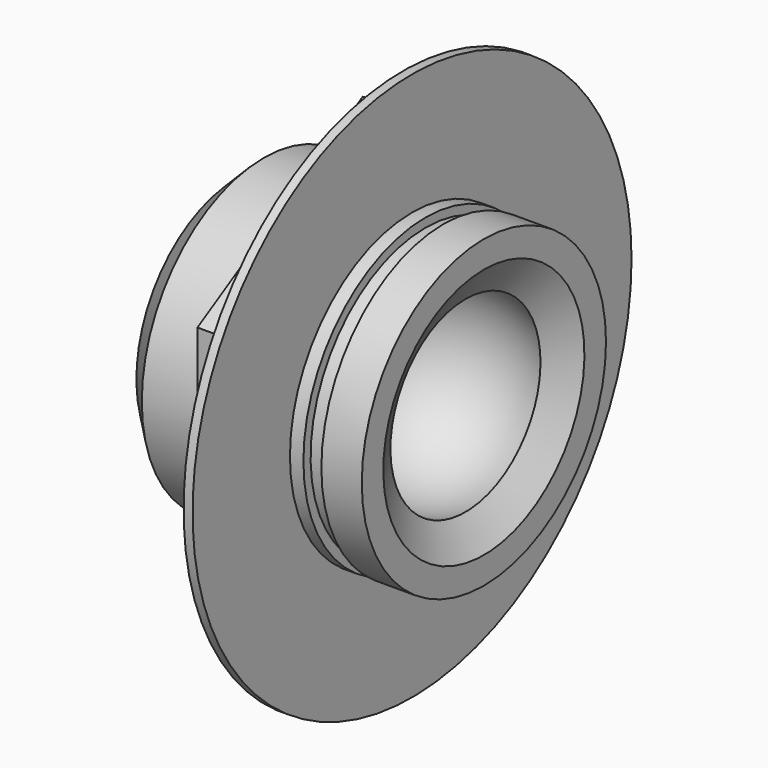
from build123d import *

# Parameters (mm, degrees)
F3_DEPTH = 25
F4_SIZE  = 3
F5_R     = 30.5581123827
F5_R_2   = 17
F6_DEPTH = 1


with BuildPart() as f1:
    # F0 (on Front) → F1 (revolve)
    with BuildSketch(Plane.XZ):
        with BuildLine():
            Line((0, 17), (0, 0))
            Line((0, 0), (11, 0))
            ThreePointArc((11, 0), (15.5551164444, 8.914228848), (25.4479047191, 10.4456667115))
            Line((25.4479047191, 10.4456667115), (27.5, 14))
            Line((27.5, 14), (27.5, 17))
            Line((27.5, 17), (23, 17))
            Line((23, 17), (23, 16))
            Line((23, 16), (21, 16))
            Line((21, 16), (21, 17))
            Line((21, 17), (18.5, 17))
            Line((18.5, 17), (18.5, 40))
            Line((18.5, 40), (14, 40))
            Line((14, 40), (14, 17))
            Line((14, 17), (0, 17))
        make_face()
    revolve(axis=Axis((11, 0, 0), (1, 0, 0)))

    # F2 (on face) → F3 (cut)
    with BuildSketch(Plane(origin=(14, 0, 0), x_dir=(0, -1, 0), z_dir=(-1, 0, 0))):
        with BuildLine():
            ThreePointArc((16.8416654415, -36.281652459), (20, -34.6410161514), (23, -32.7261363439))
            Line((23, -32.7261363439), (23, -13.2790561914))
            Line((23, -13.2790561914), (0, -26.5581123827))
            Line((0, -26.5581123827), (16.8416654415, -36.281652459))
        make_face()
        with BuildLine():
            Line((23, -13.2790561914), (23, -32.7261363439))
            ThreePointArc((23, -32.7261363439), (34.6410161514, -20), (39.8416654415, -3.5555161151))
            Line((39.8416654415, -3.5555161151), (23, -13.2790561914))
        make_face()
        with BuildLine():
            Line((23, 13.2790561914), (23, -13.2790561914))
            Line((23, -13.2790561914), (39.8416654415, -3.5555161151))
            ThreePointArc((39.8416654415, -3.5555161151), (39.9603967552, -1.7795199266), (40, 0))
            ThreePointArc((40, 0), (39.9603967552, 1.7795199266), (39.8416654415, 3.5555161151))
            Line((39.8416654415, 3.5555161151), (23, 13.2790561914))
        make_face()
        with BuildLine():
            Line((23, 32.7261363439), (23, 13.2790561914))
            Line((23, 13.2790561914), (39.8416654415, 3.5555161151))
            ThreePointArc((39.8416654415, 3.5555161151), (34.6410161514, 20), (23, 32.7261363439))
        make_face()
        with BuildLine():
            Line((0, 26.5581123827), (23, 13.2790561914))
            Line((23, 13.2790561914), (23, 32.7261363439))
            ThreePointArc((23, 32.7261363439), (20, 34.6410161514), (16.8416654415, 36.281652459))
            Line((16.8416654415, 36.281652459), (0, 26.5581123827))
        make_face()
        with BuildLine():
            Line((-16.8416654415, 36.281652459), (0, 26.5581123827))
            Line((0, 26.5581123827), (16.8416654415, 36.281652459))
            ThreePointArc((16.8416654415, 36.281652459), (0, 40), (-16.8416654415, 36.281652459))
        make_face()
        with BuildLine():
            Line((-23, 13.2790561914), (0, 26.5581123827))
            Line((0, 26.5581123827), (-16.8416654415, 36.281652459))
            ThreePointArc((-16.8416654415, 36.281652459), (-20, 34.6410161514), (-23, 32.7261363439))
            Line((-23, 32.7261363439), (-23, 13.2790561914))
        make_face()
        with BuildLine():
            Line((-39.8416654415, -3.5555161151), (-23, -13.2790561914))
            Line((-23, -13.2790561914), (-23, 13.2790561914))
            Line((-23, 13.2790561914), (-39.8416654415, 3.5555161151))
            ThreePointArc((-39.8416654415, 3.5555161151), (-40, 0), (-39.8416654415, -3.5555161151))
        make_face()
        with BuildLine():
            Line((-23, -32.7261363439), (-23, -13.2790561914))
            Line((-23, -13.2790561914), (-39.8416654415, -3.5555161151))
            ThreePointArc((-39.8416654415, -3.5555161151), (-34.6410161514, -20), (-23, -32.7261363439))
        make_face()
        with BuildLine():
            Line((-16.8416654415, -36.281652459), (0, -26.5581123827))
            Line((0, -26.5581123827), (-23, -13.2790561914))
            Line((-23, -13.2790561914), (-23, -32.7261363439))
            ThreePointArc((-23, -32.7261363439), (-20, -34.6410161514), (-16.8416654415, -36.281652459))
        make_face()
        with BuildLine():
            ThreePointArc((-16.8416654415, -36.281652459), (0, -40), (16.8416654415, -36.281652459))
            Line((16.8416654415, -36.281652459), (0, -26.5581123827))
            Line((0, -26.5581123827), (-16.8416654415, -36.281652459))
        make_face()
        with BuildLine():
            Line((-39.8416654415, 3.5555161151), (-23, 13.2790561914))
            Line((-23, 13.2790561914), (-23, 32.7261363439))
            ThreePointArc((-23, 32.7261363439), (-34.6410161514, 20), (-39.8416654415, 3.5555161151))
        make_face()
    extrude(amount=-F3_DEPTH, mode=Mode.SUBTRACT)

    # F4
    f4_edges = [f1.edges().sort_by_distance(p)[0] for p in [
        (0, 0, -17),
    ]]
    chamfer(f4_edges, length=F4_SIZE)

    # F5 (on face) → F6 (join)
    with BuildSketch(Plane.YZ.offset(18.5)):
        Circle(F5_R)
        Polygon((23, 13.2790561914), (23, -13.2790561914), (0, -26.5581123827), (-23, -13.2790561914), (-23, 13.2790561914), (0, 26.5581123827), align=None, mode=Mode.SUBTRACT)
        Polygon((0, -26.5581123827), (23, -13.2790561914), (23, 13.2790561914), (0, 26.5581123827), (-23, 13.2790561914), (-23, -13.2790561914), align=None)
        Circle(F5_R_2, mode=Mode.SUBTRACT)
    extrude(amount=F6_DEPTH)


solid = f1.part
